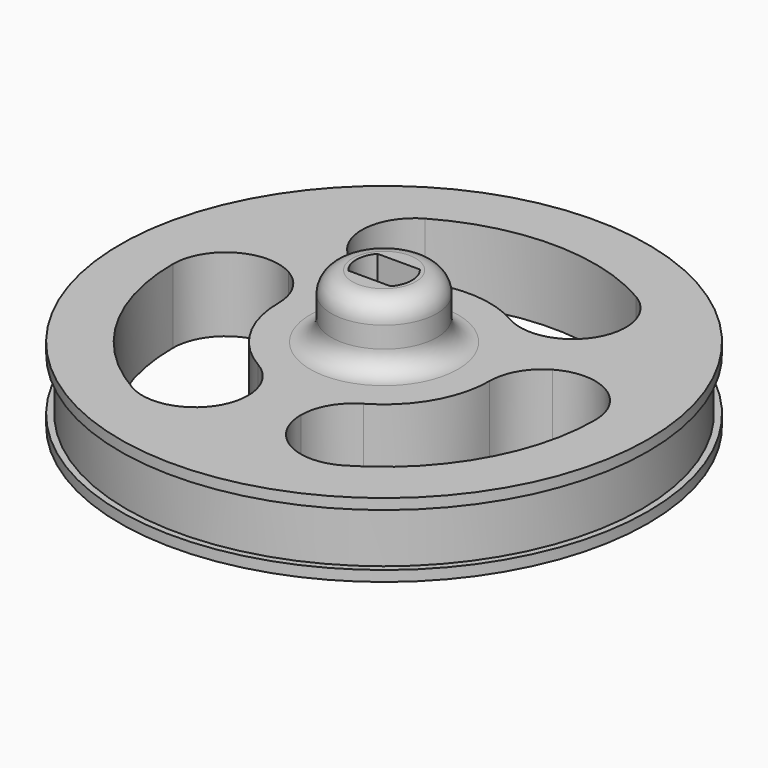
from build123d import *

# Parameters (mm, degrees)
F0_R         = 25
F1_DEPTH     = 7
F2_R         = 5
F3_DEPTH     = 6
F5_DEPTH     = 8
F7_R         = 25
F7_R_2       = 24.4
F8_DEPTH     = 5
F10_DEPTH    = 25
F11_R        = 5
F12_T1_DEPTH = 7
F13_R        = 2


# Not quite as in the source:
# - a fillet or chamfer that OpenCascade refuses, or shapes differently, is made with other operations: its cross-section is extruded or revolved along the edge and cut away or added


with BuildPart() as f1:
    # F0 (on Top) → F1 (new body)
    with BuildSketch(Plane.XY):
        Circle(F0_R)
    extrude(amount=F1_DEPTH)

    # F2 (on face) → F3 (join)
    with BuildSketch(Plane.XY.offset(7)):
        Circle(F2_R)
    extrude(amount=F3_DEPTH)

    # F4 (on face) → F5 (cut)
    with BuildSketch(Plane.XY.offset(13)):
        with BuildLine():
            Line((2.005093514, 1.725), (-2.005093514, 1.725))
            ThreePointArc((-2.005093514, 1.725), (-2.645, 0), (-2.005093514, -1.725))
            Line((-2.005093514, -1.725), (2.005093514, -1.725))
            ThreePointArc((2.005093514, -1.725), (2.645, 0), (2.005093514, 1.725))
        make_face()
    extrude(amount=-F5_DEPTH, mode=Mode.SUBTRACT)

    # F7 (on offset) → F8 (cut)
    with BuildSketch(Plane.XY.offset(1)):
        Circle(F7_R)
        Circle(F7_R_2, mode=Mode.SUBTRACT)
    extrude(amount=F8_DEPTH, mode=Mode.SUBTRACT)

    # F9 (on face) → F10 (cut)
    with BuildSketch(Plane.XY.offset(7)):
        with BuildLine():
            Line((7.1352549156, 7.0062926922), (15.9346604169, 12.0866318271))
            ThreePointArc((15.9346604169, 12.0866318271), (0, 20.0000017881), (-15.9346604169, 12.0866318271))
            Line((-15.9346604169, 12.0866318271), (-7.1352549156, 7.0062926922))
            ThreePointArc((-7.1352549156, 7.0062926922), (0, 10), (7.1352549156, 7.0062926922))
        make_face()
        with BuildLine():
            ThreePointArc((2.5, -19.8431366353), (15.0000012666, -13.2287578225), (20.0000017881, 0))
            ThreePointArc((20.0000017881, 0), (19.6047610649, 3.9564397015), (18.4346604169, 7.7565048082))
            Line((18.4346604169, 7.7565048082), (9.6352549156, 2.6761656733))
            ThreePointArc((9.6352549156, 2.6761656733), (9.9083941473, 1.3504537837), (10, 0))
            ThreePointArc((10, 0), (7.9056941504, -6.123724357), (2.5, -9.6824583655))
            Line((2.5, -9.6824583655), (2.5, -19.8431366353))
        make_face()
        with BuildLine():
            ThreePointArc((-18.4346604169, 7.7565048082), (-17.3205096243, -10.0000008941), (-2.5, -19.8431366353))
            Line((-2.5, -19.8431366353), (-2.5, -9.6824583655))
            ThreePointArc((-2.5, -9.6824583655), (-8.6602540378, -5), (-9.6352549156, 2.6761656733))
            Line((-9.6352549156, 2.6761656733), (-18.4346604169, 7.7565048082))
        make_face()
    extrude(amount=-F10_DEPTH, mode=Mode.SUBTRACT)

    # F11
    f11_edges = [f1.edges().sort_by_distance(p)[0] for p in [
        (-18.43466, 7.756505, 3.5),
        (-15.93466, 12.086632, 3.5),
        (15.93466, 12.086632, 3.5),
        (18.43466, 7.756505, 3.5),
        (2.5, -19.843137, 3.5),
        (-2.5, -19.843137, 3.5),
    ]]
    fillet(f11_edges, radius=F11_R)

    # F12: fillet of radius 5 on 6 edges, made by hand

    # F12_s2 → F12_t1 (join)
    with BuildSketch(Plane.XY):
        with BuildLine():
            ThreePointArc((-12.5, 4.3301270189), (-10.6698729811, 2.5), (-10, 0))
            ThreePointArc((-10, 0), (-9.9083941473, 1.3504537837), (-9.6352549156, 2.6761656733))
            Line((-9.6352549156, 2.6761656733), (-12.5, 4.3301270189))
        make_face()
        with BuildLine():
            ThreePointArc((-2.5, -12.9903810568), (-3.1698729811, -10.4903810568), (-5, -8.6602540378))
            ThreePointArc((-5, -8.6602540378), (-3.7846697903, -9.2561479341), (-2.5, -9.6824583655))
            Line((-2.5, -9.6824583655), (-2.5, -12.9903810568))
        make_face()
        with BuildLine():
            ThreePointArc((2.5, -12.9903810568), (3.1698729811, -10.4903810568), (5, -8.6602540378))
            ThreePointArc((5, -8.6602540378), (3.7846697903, -9.2561479341), (2.5, -9.6824583655))
            Line((2.5, -9.6824583655), (2.5, -12.9903810568))
        make_face()
        with BuildLine():
            ThreePointArc((12.5, 4.3301270189), (10.6698729811, 2.5), (10, 0))
            ThreePointArc((10, 0), (9.9083941473, 1.3504537837), (9.6352549156, 2.6761656733))
            Line((9.6352549156, 2.6761656733), (12.5, 4.3301270189))
        make_face()
        with BuildLine():
            ThreePointArc((10, 8.6602540378), (7.5, 7.9903810568), (5, 8.6602540378))
            ThreePointArc((5, 8.6602540378), (6.123724357, 7.9056941504), (7.1352549156, 7.0062926922))
            Line((7.1352549156, 7.0062926922), (10, 8.6602540378))
        make_face()
        with BuildLine():
            ThreePointArc((-10, 8.6602540378), (-7.5, 7.9903810568), (-5, 8.6602540378))
            ThreePointArc((-5, 8.6602540378), (-6.123724357, 7.9056941504), (-7.1352549156, 7.0062926922))
            Line((-7.1352549156, 7.0062926922), (-10, 8.6602540378))
        make_face()
    extrude(amount=F12_T1_DEPTH)

    # F13
    f13_edges = [f1.edges().sort_by_distance(p)[0] for p in [
        (-5, 0, 7),
        (-5, 0, 13),
    ]]
    fillet(f13_edges, radius=F13_R)


solid = f1.part
